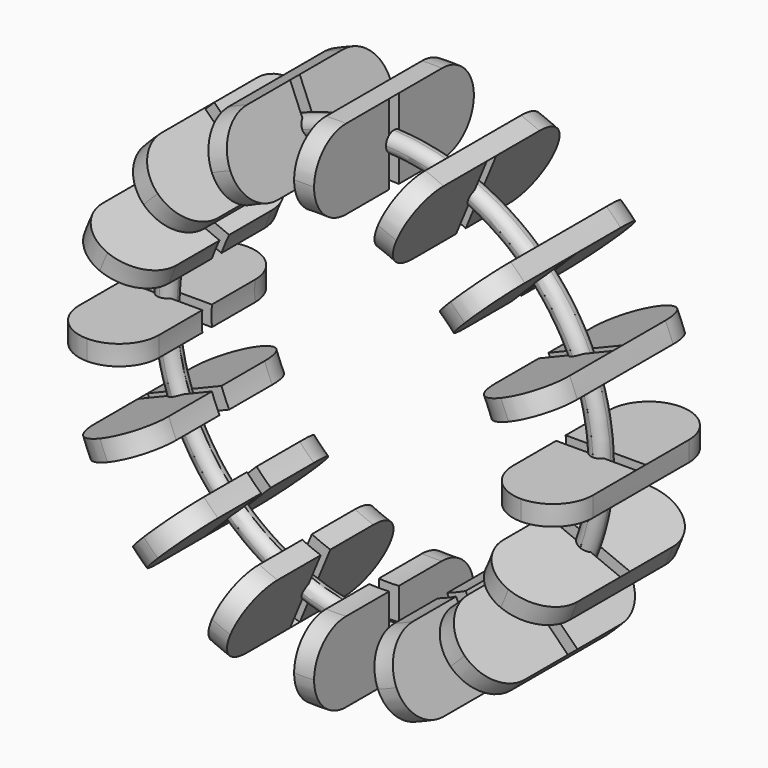
from build123d import *

# Parameters (mm, degrees)
F1_DEPTH      = 5
F1_DEPTH_BACK = 5
F2_R          = 1.99999
F3_W          = 0.6
F3_H          = 4.0043832996
F4_DEPTH      = 2
F4_DEPTH_BACK = 2
F5_START      = -0.3
F5_DEPTH      = 1.7
F6_COUNT      = 16
F7_DEPTH      = 0.5
F7_DEPTH_BACK = 0.5
F8_R          = 0.49999


# Not quite as in the source:
# - a fillet or chamfer is up to 0.001 mm smaller than in the source, because OpenCascade refuses the exact size


with BuildPart() as f1:
    # F0 (on Front) → F1 (new body, two sides)
    with BuildSketch(Plane.XZ) as f1_sk:
        with BuildLine():
            ThreePointArc((-0.5, 8.8609042992), (0, 8.875), (0.5, 8.8609042992))
            Line((0.5, 8.8609042992), (0.5, 10.3629448035))
            ThreePointArc((0.5, 10.3629448035), (0, 10.375), (-0.5, 10.3629448035))
            Line((-0.5, 10.3629448035), (-0.5, 8.8609042992))
        make_face()
        with BuildLine():
            ThreePointArc((-0.5, 11.3640056758), (0, 11.375), (0.5, 11.3640056758))
            Line((0.5, 11.3640056758), (0.5, 12.8652875988))
            ThreePointArc((0.5, 12.8652875988), (0, 12.875), (-0.5, 12.8652875988))
            Line((-0.5, 12.8652875988), (-0.5, 11.3640056758))
        make_face()
        with BuildLine():
            ThreePointArc((-0.5, 10.3629448035), (0, 10.375), (0.5, 10.3629448035))
            Line((0.5, 10.3629448035), (0.5, 11.3640056758))
            ThreePointArc((0.5, 11.3640056758), (0, 11.375), (-0.5, 11.3640056758))
            Line((-0.5, 11.3640056758), (-0.5, 10.3629448035))
        make_face()
    extrude(amount=F1_DEPTH)
    extrude(f1_sk.sketch, amount=-F1_DEPTH_BACK)

    # F2 (radius 2 in the source; OpenCascade refuses exactly that, so slightly less here)
    f2_edges = [f1.edges().sort_by_distance(p)[0] for p in [
        (0, -5, 12.875),
        (0, -5, 8.875),
        (0, 5, 12.875),
        (0, 5, 8.875),
    ]]
    fillet(f2_edges, radius=F2_R)

    # F3 (on Right) → F4 (cut, two sides)
    with BuildSketch(Plane.YZ) as f4_sk:
        with Locations((0, 10.863095949)):
            Rectangle(F3_W, F3_H)
    extrude(amount=F4_DEPTH, mode=Mode.SUBTRACT)
    extrude(f4_sk.sketch, amount=-F4_DEPTH_BACK, mode=Mode.SUBTRACT)

    # F3 (on Right) → F5 (cut)
    with BuildSketch(Plane.YZ.offset(F5_START)):
        with Locations((0, 10.863095949)):
            Rectangle(F3_W, F3_H)
    extrude(amount=-F5_DEPTH, mode=Mode.SUBTRACT)


with BuildPart() as f6_1:
    # F6: instance of F1
    add(f1.part.rotate(Axis((0, 0, 0), (0, -1, 0)), 1 * 360 / F6_COUNT))


with BuildPart() as f6_2:
    # F6: instance of F1
    add(f1.part.rotate(Axis((0, 0, 0), (0, -1, 0)), 2 * 360 / F6_COUNT))


with BuildPart() as f6_3:
    # F6: instance of F1
    add(f1.part.rotate(Axis((0, 0, 0), (0, -1, 0)), 3 * 360 / F6_COUNT))


with BuildPart() as f6_4:
    # F6: instance of F1
    add(f1.part.rotate(Axis((0, 0, 0), (0, -1, 0)), 4 * 360 / F6_COUNT))


with BuildPart() as f6_5:
    # F6: instance of F1
    add(f1.part.rotate(Axis((0, 0, 0), (0, -1, 0)), 5 * 360 / F6_COUNT))


with BuildPart() as f6_6:
    # F6: instance of F1
    add(f1.part.rotate(Axis((0, 0, 0), (0, -1, 0)), 6 * 360 / F6_COUNT))


with BuildPart() as f6_7:
    # F6: instance of F1
    add(f1.part.rotate(Axis((0, 0, 0), (0, -1, 0)), 7 * 360 / F6_COUNT))


with BuildPart() as f6_8:
    # F6: instance of F1
    add(f1.part.rotate(Axis((0, 0, 0), (0, -1, 0)), 8 * 360 / F6_COUNT))


with BuildPart() as f6_9:
    # F6: instance of F1
    add(f1.part.rotate(Axis((0, 0, 0), (0, -1, 0)), 9 * 360 / F6_COUNT))


with BuildPart() as f6_10:
    # F6: instance of F1
    add(f1.part.rotate(Axis((0, 0, 0), (0, -1, 0)), 10 * 360 / F6_COUNT))


with BuildPart() as f6_11:
    # F6: instance of F1
    add(f1.part.rotate(Axis((0, 0, 0), (0, -1, 0)), 11 * 360 / F6_COUNT))


with BuildPart() as f6_12:
    # F6: instance of F1
    add(f1.part.rotate(Axis((0, 0, 0), (0, -1, 0)), 12 * 360 / F6_COUNT))


with BuildPart() as f6_13:
    # F6: instance of F1
    add(f1.part.rotate(Axis((0, 0, 0), (0, -1, 0)), 13 * 360 / F6_COUNT))


with BuildPart() as f6_14:
    # F6: instance of F1
    add(f1.part.rotate(Axis((0, 0, 0), (0, -1, 0)), 14 * 360 / F6_COUNT))


with BuildPart() as f6_15:
    # F6: instance of F1
    add(f1.part.rotate(Axis((0, 0, 0), (0, -1, 0)), 15 * 360 / F6_COUNT))


with BuildPart() as f7:
    # F0 (on Front) → F7 (new body, two sides)
    with BuildSketch(Plane.XZ) as f7_sk:
        with BuildLine():
            Line((0.5, 11.3640056758), (0.5, 10.3629448035))
            ThreePointArc((0.5, 10.3629448035), (7.5109295363, 7.1572733984), (10.375, 0))
            ThreePointArc((10.375, 0), (-7.1572733984, -7.5109295363), (-0.5, 10.3629448035))
            Line((-0.5, 10.3629448035), (-0.5, 11.3640056758))
            ThreePointArc((-0.5, 11.3640056758), (-7.8645764349, -8.2182152868), (11.375, 0))
            ThreePointArc((11.375, 0), (8.2182152868, 7.8645764349), (0.5, 11.3640056758))
        make_face()
    extrude(amount=F7_DEPTH)
    extrude(f7_sk.sketch, amount=-F7_DEPTH_BACK)

    # F8 (radius 0.5 in the source; OpenCascade refuses exactly that, so slightly less here)
    f8_edges = [f7.edges().sort_by_distance(p)[0] for p in [
        (-7.864576, 0.5, -8.218215),
        (-7.864576, -0.5, -8.218215),
        (0, -0.5, -10.375),
        (0, 0.5, -10.375),
    ]]
    fillet(f8_edges, radius=F8_R)


solid = Compound([f1.part, f6_1.part, f6_2.part, f6_3.part, f6_4.part, f6_5.part, f6_6.part, f6_7.part, f6_8.part, f6_9.part, f6_10.part, f6_11.part, f6_12.part, f6_13.part, f6_14.part, f6_15.part, f7.part])
